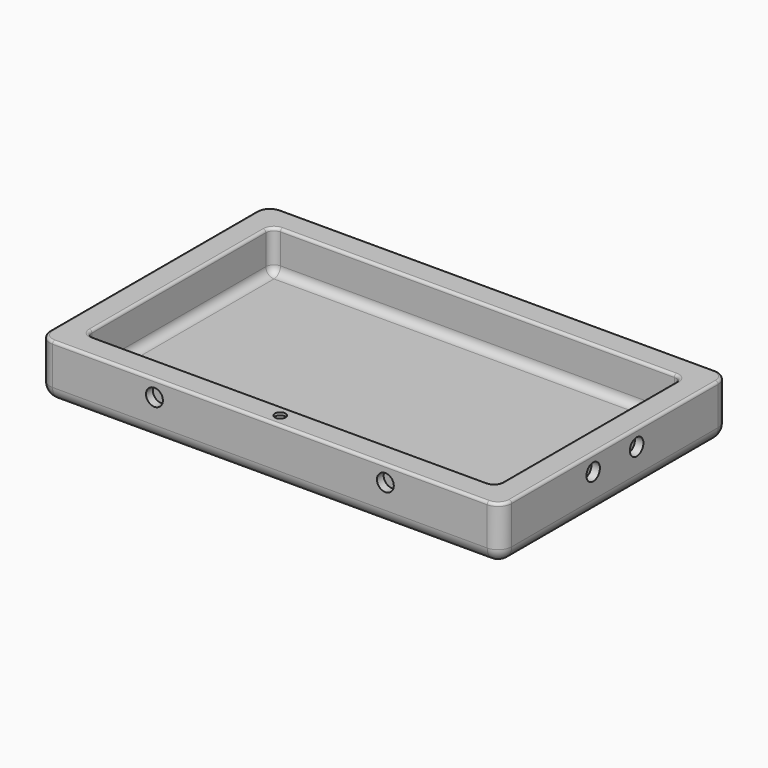
from build123d import *

# Parameters (mm, degrees)
F0_W      = 170
F0_H      = 105
F0_R      = 2
F1_DEPTH  = 20
F2_DEPTH  = 15
F3_R      = 5
F4_R      = 3
F5_R      = 1
F6_R      = 3.1
F7_DEPTH  = 3.1
F8_R      = 3.1
F9_DEPTH  = 3.1
F10_R     = 3.1
F11_DEPTH = 3.1
F12_R     = 3.1
F13_DEPTH = 3.1
F14_DEPTH = 1
F15_ANGLE = 180


# Not quite as in the source:
# - a feature names something its author has since deleted; it is built from what else it names


with BuildPart() as f1:
    # F0 (on Top) → F1 (new body)
    with BuildSketch(Plane.XY):
        Rectangle(F0_W, F0_H)
        with Locations((0, -47.75)):
            Circle(F0_R, mode=Mode.SUBTRACT)
        with BuildLine():
            ThreePointArc((-75.5, 40), (-74.6213203436, 42.1213203436), (-72.5, 43))
            Line((-72.5, 43), (72.5, 43))
            ThreePointArc((72.5, 43), (74.6213203436, 42.1213203436), (75.5, 40))
            Line((75.5, 40), (75.5, -40))
            ThreePointArc((75.5, -40), (74.6213203436, -42.1213203436), (72.5, -43))
            Line((72.5, -43), (-72.5, -43))
            ThreePointArc((-72.5, -43), (-74.6213203436, -42.1213203436), (-75.5, -40))
            Line((-75.5, -40), (-75.5, 40))
        make_face(mode=Mode.SUBTRACT)
        with BuildLine():
            Line((72.5, 43), (-72.5, 43))
            ThreePointArc((-72.5, 43), (-74.6213203436, 42.1213203436), (-75.5, 40))
            Line((-75.5, 40), (-75.5, -40))
            ThreePointArc((-75.5, -40), (-74.6213203436, -42.1213203436), (-72.5, -43))
            Line((-72.5, -43), (72.5, -43))
            ThreePointArc((72.5, -43), (74.6213203436, -42.1213203436), (75.5, -40))
            Line((75.5, -40), (75.5, 40))
            ThreePointArc((75.5, 40), (74.6213203436, 42.1213203436), (72.5, 43))
        make_face()
        with Locations((0, -47.75)):
            Circle(F0_R)
    extrude(amount=F1_DEPTH)

    # F0 (on Top) → F2 (cut)
    with BuildSketch(Plane.XY):
        with BuildLine():
            Line((72.5, 43), (-72.5, 43))
            ThreePointArc((-72.5, 43), (-74.6213203436, 42.1213203436), (-75.5, 40))
            Line((-75.5, 40), (-75.5, -40))
            ThreePointArc((-75.5, -40), (-74.6213203436, -42.1213203436), (-72.5, -43))
            Line((-72.5, -43), (72.5, -43))
            ThreePointArc((72.5, -43), (74.6213203436, -42.1213203436), (75.5, -40))
            Line((75.5, -40), (75.5, 40))
            ThreePointArc((75.5, 40), (74.6213203436, 42.1213203436), (72.5, 43))
        make_face()
    extrude(amount=F2_DEPTH, mode=Mode.SUBTRACT)

    # F3
    f3_edges = [f1.edges().sort_by_distance(p)[0] for p in [
        (0, 52.5, 20),
        (-85, 0, 20),
        (0, -52.5, 20),
        (85, 0, 20),
        (85, 52.5, 10),
        (-85, 52.5, 10),
        (-85, -52.5, 10),
        (85, -52.5, 10),
    ]]
    fillet(f3_edges, radius=F3_R)

    # F4
    f4_edges = [f1.edges().sort_by_distance(p)[0] for p in [
        (0, 43, 15),
        (-74.62132, 42.12132, 15),
        (-75.5, 0, 15),
        (-74.62132, -42.12132, 15),
        (0, -43, 15),
        (74.62132, -42.12132, 15),
        (75.5, 0, 15),
        (74.62132, 42.12132, 15),
    ]]
    fillet(f4_edges, radius=F4_R)

    # F5
    f5_edges = [f1.edges().sort_by_distance(p)[0] for p in [
        (0, 52.5, 0),
        (83.535534, 51.035534, 0),
        (-83.535534, 51.035534, 0),
        (85, 0, 0),
        (-85, 0, 0),
        (83.535534, -51.035534, 0),
        (-83.535534, -51.035534, 0),
        (0, -52.5, 0),
        (0, 43, 0),
        (-74.62132, 42.12132, 0),
        (-75.5, 0, 0),
        (-74.62132, -42.12132, 0),
        (0, -43, 0),
        (74.62132, -42.12132, 0),
        (75.5, 0, 0),
        (74.62132, 42.12132, 0),
    ]]
    fillet(f5_edges, radius=F5_R)

    # F6 (on face) → F7 (cut)
    with BuildSketch(Plane.XZ.offset(52.5)):
        with Locations((42.5, 6)):
            Circle(F6_R)
        with Locations((-42.5, 6)):
            Circle(F6_R)
    extrude(amount=-F7_DEPTH, mode=Mode.SUBTRACT)

    # F8 (on face) → F9 (cut)
    with BuildSketch(Plane(origin=(0, 52.5, 0), x_dir=(-1, 0, 0), z_dir=(0, 1, 0))):
        with Locations((42.5, 6)):
            Circle(F8_R)
        with Locations((-42.5, 6)):
            Circle(F8_R)
    extrude(amount=-F9_DEPTH, mode=Mode.SUBTRACT)

    # F10 (on face) → F11 (cut)
    with BuildSketch(Plane(origin=(-85, 0, 0), x_dir=(0, -1, 0), z_dir=(-1, 0, 0))):
        with Locations((10, 6)):
            Circle(F10_R)
        with Locations((-10, 6)):
            Circle(F10_R)
    extrude(amount=-F11_DEPTH, mode=Mode.SUBTRACT)

    # F12 (on face) → F13 (cut)
    with BuildSketch(Plane.YZ.offset(85)):
        with Locations((10, 6)):
            Circle(F12_R)
        with Locations((-10, 6)):
            Circle(F12_R)
    extrude(amount=-F13_DEPTH, mode=Mode.SUBTRACT)

    # F0 (on Top) → F14 (cut)
    with BuildSketch(Plane.XY):
        with Locations((0, -47.75)):
            Circle(F0_R)
    extrude(amount=F14_DEPTH, mode=Mode.SUBTRACT)


with BuildPart() as f1_1:
    # F15: moved
    add(f1.part.rotate(Axis((0, 0, 0), (0, 1, 0)), F15_ANGLE))


solid = f1_1.part
